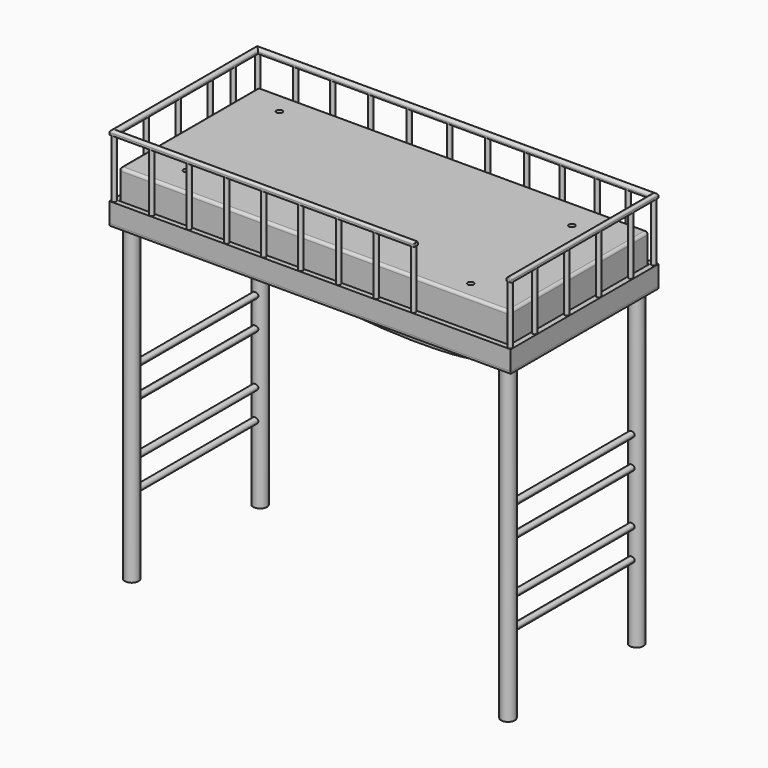
from build123d import *

# Parameters (mm, degrees)
F0_R          = 3.5
F1_DEPTH      = 160
F3_W          = 204.6981304884
F3_H          = 94.2874401808
F3_W_2        = 199.1111338139
F3_H_2        = 89.0581160784
F4_DEPTH      = 10
F5_DEPTH      = 25
F8_DEPTH      = 82.2
F7_R          = 1.5
F9_R          = 1.4243860018
F9_2_R        = 1.4243860018
F10_R         = 1.1
F11_DEPTH     = 30
F14_DEPTH     = 2.2
F15_R         = 1.1
F16_R         = 1.4002438662
F17_T1_DEPTH  = 1.7747561338
F17_T3_DEPTH  = 2.075
F17_T5_DEPTH  = 0.0043199455
F17_T8_ANGLE  = 90
F17_T10_ANGLE = 90
F17_T14_DEPTH = 4.4545638117
F17_S15_R     = 1.1
F17_T16_DEPTH = 4
F18_R         = 0.38627417
F19_DEPTH     = 1
F20_R         = 1.5
F21_DEPTH     = 4
F22_DEPTH     = 46.1


# Not quite as in the source:
# - a fillet or chamfer that OpenCascade refuses, or shapes differently, is made with other operations: its cross-section is extruded or revolved along the edge and cut away or added


with BuildPart() as f1:
    # F0 (on Top) → F1 (new body)
    with BuildSketch(Plane.XY):
        with Locations((-96.0064306855, 41.0136245191)):
            Circle(F0_R)
    extrude(amount=F1_DEPTH)


with BuildPart() as f1b:
    # F0 (on Top) → F1, piece 2 (new body)
    with BuildSketch(Plane.XY):
        with Locations((96.0138291121, 41.0175696015)):
            Circle(F0_R)
    extrude(amount=F1_DEPTH)


with BuildPart() as f1c:
    # F0 (on Top) → F1, piece 3 (new body)
    with BuildSketch(Plane.XY):
        with Locations((96.0402712226, -41.0031825304)):
            Circle(F0_R)
    extrude(amount=F1_DEPTH)


with BuildPart() as f1d:
    # F0 (on Top) → F1, piece 4 (new body)
    with BuildSketch(Plane.XY):
        with Locations((-95.9658920765, -40.9168489277)):
            Circle(F0_R)
    extrude(amount=F1_DEPTH)


with BuildPart() as f4:
    # F3 (on offset) → F4 (new body)
    with BuildSketch(Plane.XY.offset(160)):
        Rectangle(F3_W, F3_H)
        Rectangle(F3_W_2, F3_H_2, mode=Mode.SUBTRACT)
    extrude(amount=F4_DEPTH)

    # F10 (on face) → F11 (join)
    with BuildSketch(Plane.XY.offset(170)):
        with Locations((-81.666700542, -45.8517633379)):
            Circle(F10_R)
        with Locations((-62.7028048038, -45.8517633379)):
            Circle(F10_R)
        with Locations((-43.5322001576, -45.8517633379)):
            Circle(F10_R)
        with Locations((-24.5704315603, -45.8753220737)):
            Circle(F10_R)
        with Locations((-5.6567750871, -45.8753220737)):
            Circle(F10_R)
        with Locations((13.5293491185, -45.8753220737)):
            Circle(F10_R)
        with Locations((32.7726863325, -45.8753220737)):
            Circle(F10_R)
        with Locations((51.787160337, -45.8436049521)):
            Circle(F10_R)
        with Locations((101.0030061007, -45.825496316)):
            Circle(F10_R)
        with Locations((-81.666700542, 45.8266362548)):
            Circle(F10_R)
        with Locations((-62.7028048038, 45.8266362548)):
            Circle(F10_R)
        with Locations((-43.5322001576, 45.8266362548)):
            Circle(F10_R)
        with Locations((-23.8501671702, 45.8852611482)):
            Circle(F10_R)
        with Locations((-3.1968329567, 45.7855984569)):
            Circle(F10_R)
        with Locations((16.1913055927, 45.8925105631)):
            Circle(F10_R)
        with Locations((36.1218415201, 45.8208248019)):
            Circle(F10_R)
        with Locations((54.1482307017, 45.8208248019)):
            Circle(F10_R)
        with Locations((72.0514804125, 45.8132624626)):
            Circle(F10_R)
        with Locations((87.9804119468, 45.8620563149)):
            Circle(F10_R)
        with Locations((100.9320393205, 45.7421280444)):
            Circle(F10_R)
        with Locations((100.971840322, 31.0528520495)):
            Circle(F10_R)
        with Locations((101.0089591146, 10.5716679245)):
            Circle(F10_R)
        with Locations((100.9764149785, -9.6243461594)):
            Circle(F10_R)
        with Locations((100.936613977, -30.2131436765)):
            Circle(F10_R)
        with Locations((-101.0323278606, 30.1297754049)):
            Circle(F10_R)
        with Locations((-100.992526859, 15.44049941)):
            Circle(F10_R)
        with Locations((-100.9554080665, -5.0406847149)):
            Circle(F10_R)
        with Locations((-100.9879522026, -25.2366987988)):
            Circle(F10_R)
        with Locations((-101.0277532041, -45.825496316)):
            Circle(F10_R)
        with Locations((-101.0323278606, 45.8266362548)):
            Circle(F10_R)
    extrude(amount=F11_DEPTH)

    # F13 (on offset) → F14 (join)
    with BuildSketch(Plane.XY.offset(199.67)):
        Polygon((-102.3500619592, 46.9943657517), (-102.3500619592, -46.9943657517), (53.0928149819, -46.9943657517), (53.0928149819, -44.4876775146), (-99.8454981475, -44.4876775146), (-99.8454981475, 44.4876775146), (99.8454981475, 44.4876775146), (99.8454981475, -44.4876775146), (99.8454981475, -46.9943657517), (102.3500619592, -46.9943657517), (102.3500619592, 46.9943657517), align=None)
    extrude(amount=F14_DEPTH)

    # F15
    f15_edges = [f4.edges().sort_by_distance(p)[0] for p in [
        (0, 46.994366, 201.87),
        (102.350062, 0, 201.87),
        (-24.628623, -46.994366, 201.87),
        (-102.350062, 0, 201.87),
    ]]
    fillet(f15_edges, radius=F15_R)

    # F16
    f16_edges = [f4.edges().sort_by_distance(p)[0] for p in [
        (99.845498, -1.253344, 201.87),
        (0, 44.487678, 201.87),
        (-99.845498, 0, 201.87),
        (-23.376342, -44.487678, 201.87),
    ]]
    fillet(f16_edges, radius=F16_R)

    # F17: fillet of radius 0.39 on 6 edges, made by hand

    # F17_s2 → F17_t1 (cut)
    with BuildSketch(Plane.XY.offset(198.695)):
        with BuildLine():
            ThreePointArc((100.2354981475, -46.9943657517), (99.9597265029, -46.8801373964), (99.8454981475, -46.6043657517))
            Line((99.8454981475, -46.6043657517), (99.8454981475, -46.9943657517))
            Line((99.8454981475, -46.9943657517), (100.2354981475, -46.9943657517))
        make_face()
    extrude(amount=F17_T1_DEPTH, mode=Mode.SUBTRACT)

    # F17_s4 → F17_t3 (cut)
    with BuildSketch(Plane.XY.offset(198.695)):
        with BuildLine():
            ThreePointArc((101.9600619592, -46.9943657517), (102.2358336039, -46.8801373964), (102.3500619592, -46.6043657517))
            Line((102.3500619592, -46.6043657517), (102.3500619592, -46.9943657517))
            Line((102.3500619592, -46.9943657517), (101.9600619592, -46.9943657517))
        make_face()
    extrude(amount=F17_T3_DEPTH, mode=Mode.SUBTRACT)

    # F17_s6 → F17_t5 (cut)
    with BuildSketch(Plane.YZ.offset(101.2457420137)):
        with BuildLine():
            ThreePointArc((-46.9943657517, 201.48), (-46.8801373964, 201.7557716447), (-46.6043657517, 201.87))
            Line((-46.6043657517, 201.87), (-46.9943657517, 201.87))
            Line((-46.9943657517, 201.87), (-46.9943657517, 201.48))
        make_face()
    extrude(amount=F17_T5_DEPTH, mode=Mode.SUBTRACT)

    # F17_s7 → F17_t8 (revolve, cut)
    with BuildSketch(Plane.XY.offset(200.77)):
        with BuildLine():
            ThreePointArc((101.9600619592, -46.9943657517), (102.2358336039, -46.8801373964), (102.3500619592, -46.6043657517))
            Line((102.3500619592, -46.6043657517), (102.3500619592, -46.9943657517))
            Line((102.3500619592, -46.9943657517), (101.9600619592, -46.9943657517))
        make_face()
    revolve(axis=Axis((101.2500619592, -46.9943657517, 200.77), (0, -1, 0)), revolution_arc=F17_T8_ANGLE, mode=Mode.SUBTRACT)

    # F17_s9 → F17_t10 (revolve, cut)
    with BuildSketch(Plane.YZ.offset(101.2457420137)):
        with BuildLine():
            ThreePointArc((-46.9943657517, 201.48), (-46.8801373964, 201.7557716447), (-46.6043657517, 201.87))
            Line((-46.6043657517, 201.87), (-46.9943657517, 201.87))
            Line((-46.9943657517, 201.87), (-46.9943657517, 201.48))
        make_face()
    revolve(axis=Axis((101.2457420137, -46.9943657517, 200.4697561338), (0, -1, 0)), revolution_arc=F17_T10_ANGLE, mode=Mode.SUBTRACT)


with BuildPart() as f5:
    # F3 (on offset) → F5 (new body)
    with BuildSketch(Plane.XY.offset(160)):
        Rectangle(F3_W_2, F3_H_2)
    extrude(amount=F5_DEPTH)

    # F9
    f9_edges = [f5.edges().sort_by_distance(p)[0] for p in [
        (0, -44.529058, 185),
        (-99.555567, 0, 185),
        (-99.555567, -44.529058, 172.5),
        (-99.555567, 44.529058, 172.5),
        (0, 44.529058, 185),
        (99.555567, 44.529058, 172.5),
        (99.555567, 0, 185),
        (99.555567, -44.529058, 172.5),
    ]]
    fillet(f9_edges, radius=F9_R)

    # F20 (on face) → F22 (cut)
    with BuildSketch(Plane(origin=(0, 0, 159), x_dir=(1, 0, 0), z_dir=(0, 0, -1))):
        with Locations((-76.9297033548, 29.9432370812)):
            Circle(F20_R)
        with Locations((-79.7456651926, -32.9826027155)):
            Circle(F20_R)
        with Locations((72.6410150528, -28.9752800018)):
            Circle(F20_R)
        with Locations((72.4244043231, 35.2502353489)):
            Circle(F20_R)
    extrude(amount=-F22_DEPTH, mode=Mode.SUBTRACT)


with BuildPart() as f8:
    # F7 (on offset) → F8 (new body)
    with BuildSketch(Plane.XZ.offset(-41.4)):
        with BuildLine():
            ThreePointArc((96.0562303662, 93.9026201367), (97.116890538, 94.341959965), (97.5562303662, 95.4026201367))
            ThreePointArc((97.5562303662, 95.4026201367), (94.9955701945, 96.4632803085), (96.0562303662, 93.9026201367))
        make_face()
    extrude(amount=F8_DEPTH)


with BuildPart() as f8b:
    # F7 (on offset) → F8, piece 2 (new body)
    with BuildSketch(Plane.XZ.offset(-41.4)):
        with BuildLine():
            ThreePointArc((97.5562303662, 80.4026201367), (97.116890538, 81.4632803085), (96.0562303662, 81.9026201367))
            ThreePointArc((96.0562303662, 81.9026201367), (94.9955701945, 79.341959965), (97.5562303662, 80.4026201367))
        make_face()
    extrude(amount=F8_DEPTH)


with BuildPart() as f8c:
    # F7 (on offset) → F8, piece 3 (new body)
    with BuildSketch(Plane.XZ.offset(-41.4)):
        with BuildLine():
            ThreePointArc((-95.8968475461, 93.9026201367), (-94.8361873743, 94.341959965), (-94.3968475461, 95.4026201367))
            ThreePointArc((-94.3968475461, 95.4026201367), (-96.9575077179, 96.4632803085), (-95.8968475461, 93.9026201367))
        make_face()
    extrude(amount=F8_DEPTH)


with BuildPart() as f8d:
    # F7 (on offset) → F8, piece 4 (new body)
    with BuildSketch(Plane.XZ.offset(-41.4)):
        with BuildLine():
            ThreePointArc((-94.3968475461, 80.4026201367), (-94.8361873743, 81.4632803085), (-95.8968475461, 81.9026201367))
            ThreePointArc((-95.8968475461, 81.9026201367), (-96.9575077179, 79.341959965), (-94.3968475461, 80.4026201367))
        make_face()
    extrude(amount=F8_DEPTH)

    # F9#2
    f9_2_edges = [f8d.edges().sort_by_distance(p)[0] for p in [
        (-97.396848, 41.4, 80.40262),
    ]]
    fillet(f9_2_edges, radius=F9_2_R)


with BuildPart() as f8e:
    # F7 (on offset) → F8, piece 5 (new body)
    with BuildSketch(Plane.XZ.offset(-41.4)):
        with BuildLine():
            ThreePointArc((96.0562303662, 52.6505025327), (97.116890538, 53.0898423609), (97.5562303662, 54.1505025327))
            ThreePointArc((97.5562303662, 54.1505025327), (94.9955701945, 55.2111627045), (96.0562303662, 52.6505025327))
        make_face()
    extrude(amount=F8_DEPTH)


with BuildPart() as f8f:
    # F7 (on offset) → F8, piece 6 (new body)
    with BuildSketch(Plane.XZ.offset(-41.4)):
        with BuildLine():
            ThreePointArc((97.5562303662, 39.1505025327), (97.116890538, 40.2111627045), (96.0562303662, 40.6505025327))
            ThreePointArc((96.0562303662, 40.6505025327), (94.9955701945, 38.0898423609), (97.5562303662, 39.1505025327))
        make_face()
    extrude(amount=F8_DEPTH)


with BuildPart() as f8g:
    # F7 (on offset) → F8, piece 7 (new body)
    with BuildSketch(Plane.XZ.offset(-41.4)):
        with Locations((-95.8968475461, 54.1505025327)):
            Circle(F7_R)
    extrude(amount=F8_DEPTH)


with BuildPart() as f8h:
    # F7 (on offset) → F8, piece 8 (new body)
    with BuildSketch(Plane.XZ.offset(-41.4)):
        with Locations((-95.8968475461, 39.1505025327)):
            Circle(F7_R)
    extrude(amount=F8_DEPTH)


with BuildPart() as f17_tool12:
    # F17_s13 → F17_t14 (new body)
    with BuildSketch(Plane.YZ.offset(98.8704981475)):
        with BuildLine():
            ThreePointArc((-46.9943657517, 200.06), (-46.8801373964, 199.7842283553), (-46.6043657517, 199.67))
            Line((-46.6043657517, 199.67), (-46.9943657517, 199.67))
            Line((-46.9943657517, 199.67), (-46.9943657517, 200.06))
        make_face()
    extrude(amount=F17_T14_DEPTH)

    # F17_s15 → F17_t16 (cut, symmetric)
    with BuildSketch(Plane.XY.offset(199.9)):
        with Locations((101.0030061007, -45.825496316)):
            Circle(F17_S15_R)
    extrude(amount=F17_T16_DEPTH, both=True, mode=Mode.SUBTRACT)


with BuildPart() as f4_1:
    add(f4.part)

    # F17_t11: cut F17_tool12
    add(f17_tool12.part, mode=Mode.SUBTRACT)

    # F18
    f18_edges = [f4_1.edges().sort_by_distance(p)[0] for p in [
        (53.092815, -45.741022, 199.67),
        (53.092815, -46.672183, 201.547817),
        (53.092815, -44.897799, 201.459878),
        (53.092815, -44.487678, 200.069878),
        (53.092815, -46.994366, 200.22),
        (53.092815, -45.891144, 201.87),
    ]]
    fillet(f18_edges, radius=F18_R)


with BuildPart() as f19:
    # F3 (on offset) → F19 (new body)
    with BuildSketch(Plane.XY.offset(160)):
        Rectangle(F3_W, F3_H)
        Rectangle(F3_W_2, F3_H_2, mode=Mode.SUBTRACT)
        Rectangle(F3_W_2, F3_H_2)
    extrude(amount=-F19_DEPTH)


with BuildPart() as f21:
    # F20 (on face) → F21 (new body)
    with BuildSketch(Plane(origin=(0, 0, 159), x_dir=(1, 0, 0), z_dir=(0, 0, -1))):
        with BuildLine():
            add(Edge.make_bspline(
                [(79.4879347086, 39.8664809763), (69.8542323002, 45.131009936), (2.3599866869, 42.5748234443), (-37.6307216943, 24.3331480172), (-97.0130873513, 59.065156732), (-90.4916904353, -42.8681123511), (-75.749666066, -36.8836700597), (65.6016553877, -37.7584637196), (85.8579272776, -36.3728638924), (80.8870730611, 26.7035363158), (83.6803913962, 37.5754293424), (79.4879347086, 39.8664809763)],
                knots=[0, 0, 0, 0, 0.1381184316, 0.2547924483, 0.3592794302, 0.4982120953, 0.5539963423, 0.7484958868, 0.8159477874, 0.939892731, 1, 1, 1, 1], degree=3))
        make_face()
        with Locations((-79.7456651926, -32.9826027155)):
            Circle(F20_R, mode=Mode.SUBTRACT)
        with Locations((72.6410150528, -28.9752800018)):
            Circle(F20_R, mode=Mode.SUBTRACT)
        with Locations((-76.9297033548, 29.9432370812)):
            Circle(F20_R, mode=Mode.SUBTRACT)
        with Locations((72.4244043231, 35.2502353489)):
            Circle(F20_R, mode=Mode.SUBTRACT)
    extrude(amount=F21_DEPTH)


solid = Compound([f1.part, f1b.part, f1c.part, f1d.part, f5.part, f8.part, f8b.part, f8c.part, f8d.part, f8e.part, f8f.part, f8g.part, f8h.part, f4_1.part, f19.part, f21.part])
